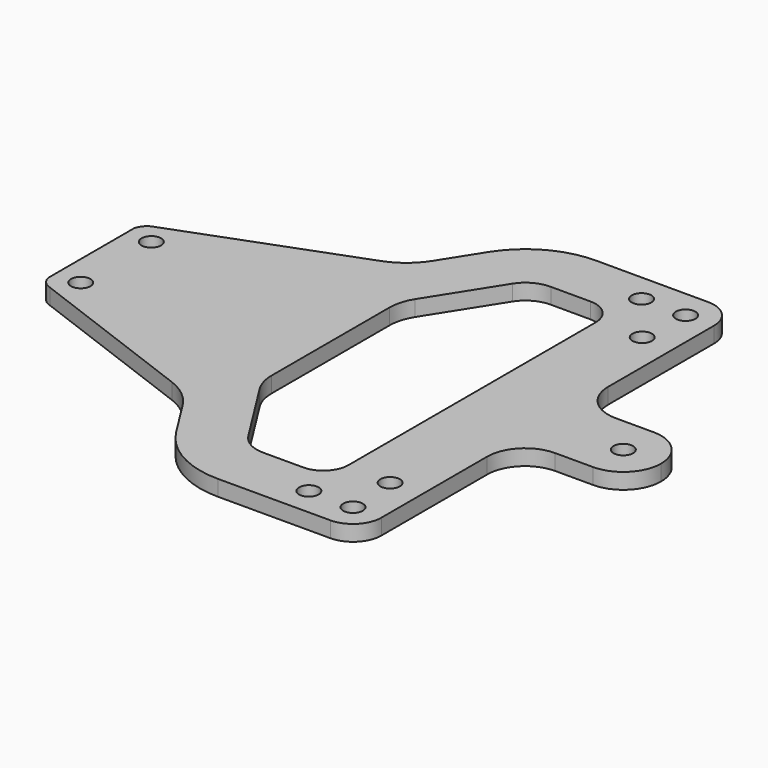
from build123d import *

# Parameters (mm, degrees)
F0_R     = 1.55
F1_DEPTH = 2.5


# Not quite as in the source:
# - ends of sketch curves that miss each other by under 0.0002 mm in the source are joined


with BuildPart() as f1:
    # F0 (on Top) → F1 (new body)
    with BuildSketch(Plane.XY):
        with BuildLine():
            Line((24.1317584196, 12.0030992724), (24.1317584196, 33.007258608))
            ThreePointArc((24.1317584196, 33.007258608), (22.8094861978, 36.1776713218), (19.6355297089, 37.4914143753))
            Line((19.6355297089, 37.4914143753), (1.8379933168, 37.5062195629))
            ThreePointArc((1.8379933168, 37.5062195629), (-4.952633867, 35.7733094677), (-10.0545165801, 30.9684798423))
            Line((-10.0545165801, 30.9684798423), (-13.9594315472, 24.7955182975))
            ThreePointArc((-13.9594315472, 24.7955182975), (-16.1001567778, 22.383955311), (-18.8970513925, 20.7790499976))
            Line((-18.8970513925, 20.7790499976), (-46.5253097099, 10.4110515716))
            ThreePointArc((-46.5253097099, 10.4110515716), (-47.6965598622, 9.7014043841), (-48.3182136925, 8.4811697487))
            Line((-48.3182136925, 8.4811697487), (-48.3182136925, -8.4811697487))
            ThreePointArc((-48.3182136925, -8.4811697487), (-47.6965598622, -9.7014043841), (-46.5253097099, -10.4110515716))
            Line((-46.5253097099, -10.4110515716), (-18.8970513925, -20.7790499976))
            ThreePointArc((-18.8970513925, -20.7790499976), (-16.1001567778, -22.383955311), (-13.9594315472, -24.7955182975))
            Line((-13.9594315472, -24.7955182975), (-10.0545165801, -30.9684798423))
            ThreePointArc((-10.0545165801, -30.9684798423), (-4.952633867, -35.7733094677), (1.8379933168, -37.5062195629))
            Line((1.8379933168, -37.5062195629), (19.635501821, -37.4914143985))
            ThreePointArc((19.635501821, -37.4914143985), (22.8150621521, -36.1720727032), (24.1317584196, -32.9914159555))
            Line((24.1317584196, -32.9914159555), (24.1317584196, -12.0030992724))
            Line((24.1317584196, -12.0030992724), (24.1317584196, -12))
            ThreePointArc((24.1317584196, -12), (25.8891177325, -7.7573593129), (30.1317584196, -6))
            Line((30.1317584196, -6), (36.1317584196, -6))
            ThreePointArc((36.1317584196, -6), (40.3733032071, -4.2437363038), (42.1317576192, -0.003099272))
            Line((42.1317576192, -0.003099272), (42.1317584196, 0))
            ThreePointArc((42.1317584196, 0), (40.3743991067, 4.2426406871), (36.1317584196, 6))
            Line((36.1317584196, 6), (30.1317584196, 6))
            ThreePointArc((30.1317584196, 6), (25.8891177325, 7.7573593129), (24.1317584196, 12))
            Line((24.1317584196, 12), (24.1317584196, 12.0030992724))
        make_face()
        with Locations((-44.3682136925, -7)):
            Circle(F0_R, mode=Mode.SUBTRACT)
        with Locations((12.6317863075, -32.997239003)):
            Circle(F0_R, mode=Mode.SUBTRACT)
        with Locations((19.1317584196, -25)):
            Circle(F0_R, mode=Mode.SUBTRACT)
        with Locations((19.6317863075, -32.9914159323)):
            Circle(F0_R, mode=Mode.SUBTRACT)
        with Locations((-44.3682136925, 7)):
            Circle(F0_R, mode=Mode.SUBTRACT)
        with BuildLine():
            Line((-9.2339508783, 15.4306240067), (-2.4342503505, 26.1797159146))
            ThreePointArc((-2.4342503505, 26.1797159146), (-0.5889861734, 27.9038009834), (1.8634800061, 28.5061952445))
            Line((1.8634800061, 28.5061952445), (8.1350890009, 28.5009780993))
            ThreePointArc((8.1350890009, 28.5009780993), (10.9631282223, 27.3264639859), (12.1317584196, 24.4959882833))
            Line((12.1317584196, 24.4959882833), (12.1317584196, -24.5019407212))
            ThreePointArc((12.1317584196, -24.5019407212), (10.9611450551, -27.3294080096), (8.1344727862, -28.5019398002))
            Line((8.1344727862, -28.5019398002), (1.8634800061, -28.5061952445))
            ThreePointArc((1.8634800061, -28.5061952445), (-0.5889861734, -27.9038009834), (-2.4342503505, -26.1797159146))
            Line((-2.4342503505, -26.1797159146), (-9.2339508783, -15.4306240067))
            ThreePointArc((-9.2339508783, -15.4306240067), (-10.0416860208, -13.6364803831), (-10.3182136925, -11.688424981))
            Line((-10.3182136925, -11.688424981), (-10.3182136925, 11.688424981))
            ThreePointArc((-10.3182136925, 11.688424981), (-10.0416860208, 13.6364803831), (-9.2339508783, 15.4306240067))
        make_face(mode=Mode.SUBTRACT)
        with Locations((36.1317584196, 0)):
            Circle(F0_R, mode=Mode.SUBTRACT)
        with Locations((19.1317584196, 25)):
            Circle(F0_R, mode=Mode.SUBTRACT)
        with Locations((12.6317863075, 32.997239003)):
            Circle(F0_R, mode=Mode.SUBTRACT)
        with Locations((19.6317863075, 32.9914159323)):
            Circle(F0_R, mode=Mode.SUBTRACT)
    extrude(amount=F1_DEPTH)


solid = f1.part
